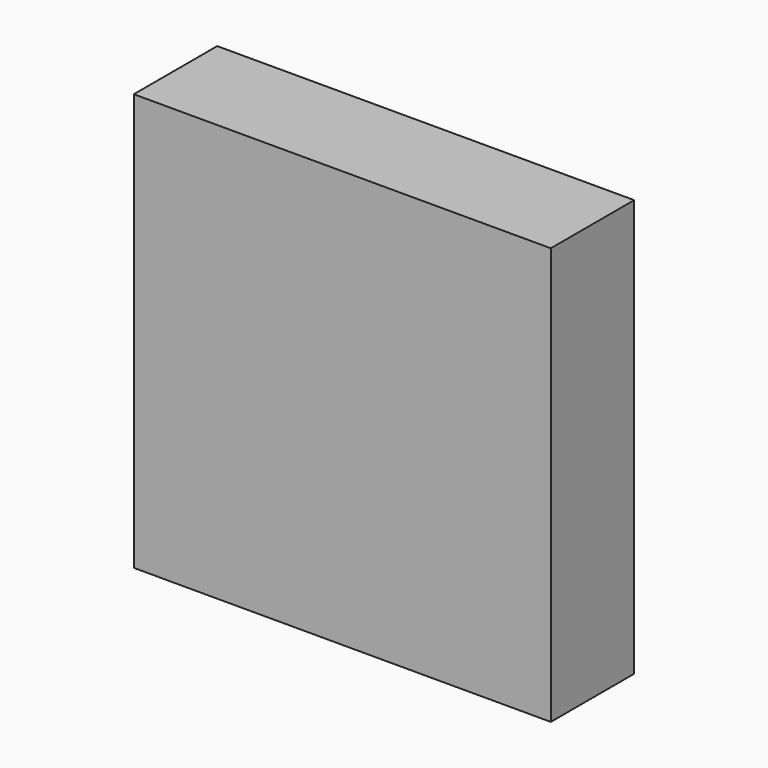
from build123d import *

# Parameters (mm, degrees)
F0_W     = 80
F0_H     = 80
F1_DEPTH = 20
F3_DEPTH = 10
F5_DEPTH = 5
F7_D     = 8
F7_DEPTH = 15
F7_TIP   = 2.4034424761


with BuildPart() as f1:
    # F0 (on Front) → F1 (new body)
    with BuildSketch(Plane.XZ):
        Rectangle(F0_W, F0_H)
    extrude(amount=F1_DEPTH)

    # F2 (on face) → F3 (cut)
    with BuildSketch(Plane(origin=(0, 0, 0), x_dir=(-1, 0, 0), z_dir=(0, 1, 0))):
        with BuildLine():
            ThreePointArc((-35, -15), (-32.0710678119, -22.0710678119), (-25, -25))
            Line((-25, -25), (15, -25))
            ThreePointArc((15, -25), (22.0710678119, -22.0710678119), (25, -15))
            Line((25, -15), (25, 25))
            ThreePointArc((25, 25), (22.0710678119, 32.0710678119), (15, 35))
            Line((15, 35), (-25, 35))
            ThreePointArc((-25, 35), (-32.0710678119, 32.0710678119), (-35, 25))
            Line((-35, 25), (-35, -15))
        make_face()
    extrude(amount=-F3_DEPTH, mode=Mode.SUBTRACT)

    # F4 (on face) → F5 (cut)
    with BuildSketch(Plane(origin=(0, -10, 0), x_dir=(-1, 0, 0), z_dir=(0, 1, 0))):
        with BuildLine():
            ThreePointArc((-25, -9), (-23.2426406871, -13.2426406871), (-19, -15))
            Line((-19, -15), (9, -15))
            ThreePointArc((9, -15), (13.2426406871, -13.2426406871), (15, -9))
            Line((15, -9), (15, 19))
            ThreePointArc((15, 19), (13.2426406871, 23.2426406871), (9, 25))
            Line((9, 25), (-19, 25))
            ThreePointArc((-19, 25), (-23.2426406871, 23.2426406871), (-25, 19))
            Line((-25, 19), (-25, -9))
        make_face()
    extrude(amount=-F5_DEPTH, mode=Mode.SUBTRACT)

    # F7
    with Locations(Plane(origin=(0, 0, 0), x_dir=(-1, 0, 0), z_dir=(0, 1, 0))):
        with Locations((-25, -32), (15, -32)):
            Hole(F7_D / 2, depth=F7_DEPTH)
            with Locations((0, 0, -(F7_DEPTH + F7_TIP / 2))):  # 118° drill point
                Cone(0, F7_D / 2, F7_TIP, mode=Mode.SUBTRACT)


solid = f1.part
